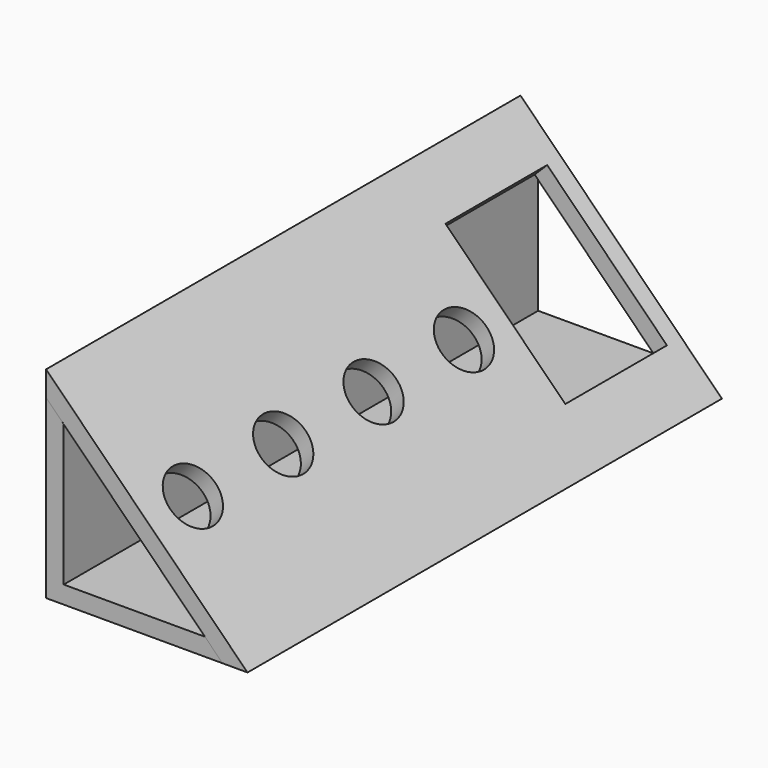
from build123d import *

# Parameters (mm, degrees)
F1_DEPTH = 533.4
F3_R     = 25.4
F3_W     = 152.4
F3_H     = 114.3
F4_DEPTH = 17.78


# Not quite as in the source:
# - a feature names something its author has since deleted; it is built from what else it names


with BuildPart() as f1:
    # F0 (on Front) → F1 (new body)
    with BuildSketch(Plane.XZ):
        Polygon((0, 158.7081573489), (0, 0), (158.75, 0), (142.8708146317, 15.875), (15.875, 15.875), (15.875, 142.837341614), align=None)
    extrude(amount=-F1_DEPTH)


with BuildPart() as f1b:
    # F0 (on Front) → F1, piece 2 (new body)
    with BuildSketch(Plane.XZ):
        Polygon((142.875, 15.875), (158.75, 0), (181.2036, 0), (0, 181.1558391243), (0, 158.75), (15.875, 142.875), (15.875, 142.837341614), (142.8708146317, 15.875), align=None)
    extrude(amount=-F1_DEPTH)

    # F3 (on face) → F4 (cut)
    with BuildSketch(Plane(origin=(90.577916415, 0, 90.601796852), x_dir=(0.7071999754, 0, -0.7070135747), z_dir=(0.7070135747, 0, 0.7071999754))):
        with Locations((1.1471814675, 50.8)):
            Circle(F3_R)
        with Locations((1.1471814675, 152.4)):
            Circle(F3_R)
        with Locations((1.1471814675, 254)):
            Circle(F3_R)
        with Locations((1.1471814675, 355.6)):
            Circle(F3_R)
        with Locations((0, 460.375)):
            Rectangle(F3_W, F3_H)
    extrude(amount=-F4_DEPTH, mode=Mode.SUBTRACT)


solid = Compound([f1.part, f1b.part])
